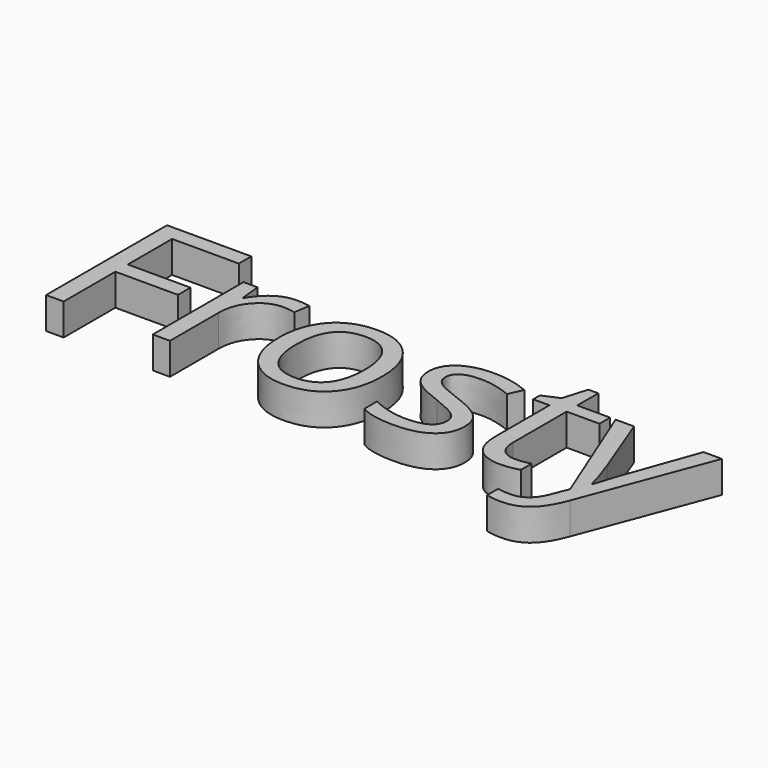
from build123d import *

# Parameters (mm, degrees)
F0_TEXT_SIZE = 33.9159302207
F1_DEPTH     = 5.08


# Not quite as in the source:
# - Text() gives the source's letters only with a copy of the font that has no kerning and outlines rounded to 1/6400 em; it was checked with that copy


with BuildPart() as f1:
    # F0 (on Top) → F1 (new body)
    with BuildSketch(Plane.XY):
        with Locations((-49.6199317276, -19.4916315377)):
            Text('Frosty', F0_TEXT_SIZE, font='Open Sans', text_align=(TextAlign.LEFT, TextAlign.BOTTOM))
    extrude(amount=F1_DEPTH)


solid = f1.part
